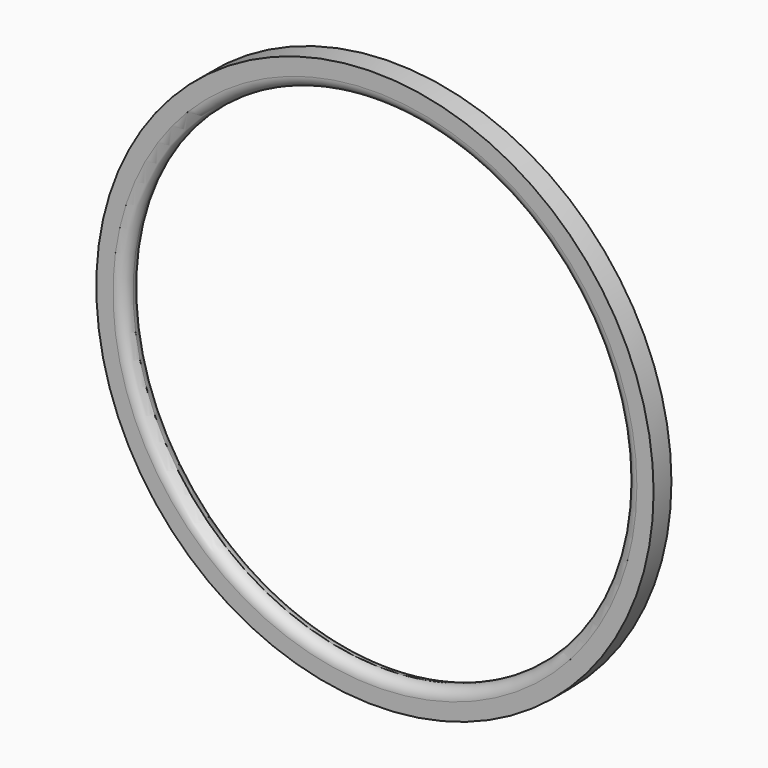
from build123d import *

# Parameters (mm, degrees)
F0_R     = 63.5
F0_R_2   = 57.15
F1_DEPTH = 5.08
F2_R     = 2.53999


# Not quite as in the source:
# - a fillet or chamfer is up to 0.001 mm smaller than in the source, because OpenCascade refuses the exact size


with BuildPart() as f1:
    # F0 (on Front) → F1 (new body)
    with BuildSketch(Plane.XZ):
        Circle(F0_R)
        Circle(F0_R_2, mode=Mode.SUBTRACT)
    extrude(amount=F1_DEPTH)

    # F2 (radius 2.54 in the source; OpenCascade refuses exactly that, so slightly less here)
    f2_edges = [f1.edges().sort_by_distance(p)[0] for p in [
        (-57.15, -5.08, 0),
        (-57.15, 0, 0),
    ]]
    fillet(f2_edges, radius=F2_R)


solid = f1.part
